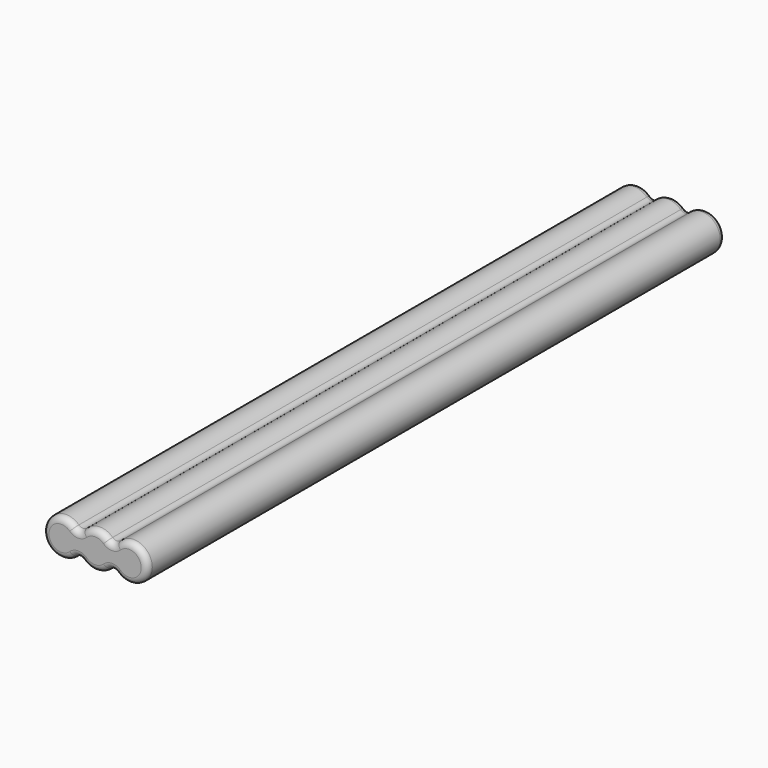
from build123d import *

# Parameters (mm, degrees)
F1_DEPTH = 74.6125
F2_R     = 1.27


with BuildPart() as f1:
    # F0 (on Front) → F1 (new body, symmetric)
    with BuildSketch(Plane.XZ):
        with BuildLine():
            ThreePointArc((3.4925, 1.5226765087), (0, 3.81), (-3.4925, 1.5226765087))
            ThreePointArc((-3.4925, 1.5226765087), (-10.795, 0), (-3.4925, -1.5226765087))
            ThreePointArc((-3.4925, -1.5226765087), (0, -3.81), (3.4925, -1.5226765087))
            ThreePointArc((3.4925, -1.5226765087), (10.795, 0), (3.4925, 1.5226765087))
        make_face()
    extrude(amount=F1_DEPTH, both=True)

    # F2
    f2_edges = [f1.edges().sort_by_distance(p)[0] for p in [
        (3.4925, 0, 1.522677),
        (-3.4925, 0, 1.522677),
        (-3.4925, 0, -1.522677),
        (3.4925, 0, -1.522677),
        (0, -74.6125, 3.81),
        (0, 74.6125, 3.81),
        (10.795, 74.6125, 0),
        (10.795, -74.6125, 0),
        (0, 74.6125, -3.81),
        (0, -74.6125, -3.81),
        (-10.795, 74.6125, 0),
        (-10.795, -74.6125, 0),
    ]]
    fillet(f2_edges, radius=F2_R)


solid = f1.part
